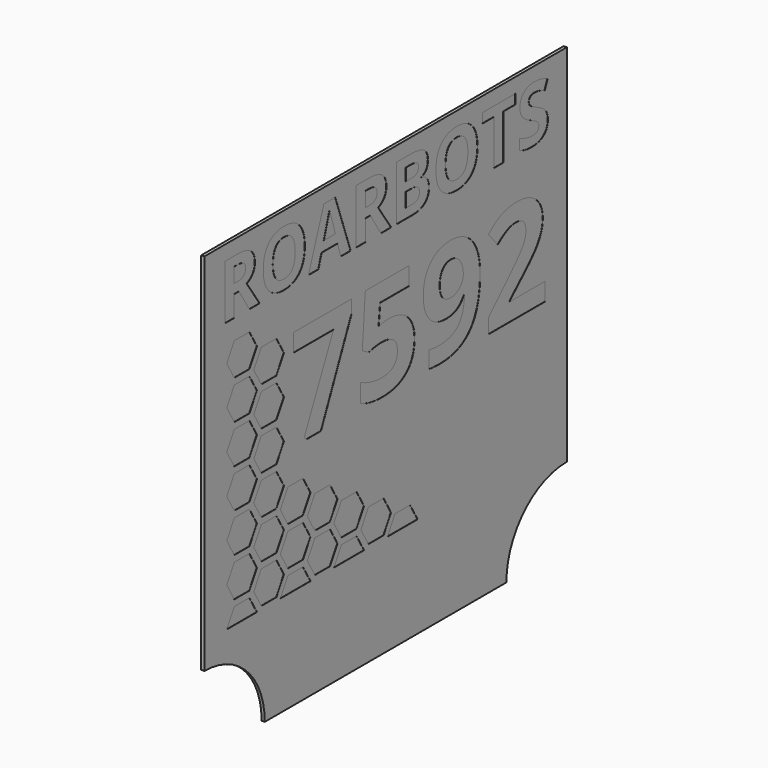
from build123d import *

# Parameters (mm, degrees)
F1_DEPTH     = 3.175
F2_TEXT_SIZE = 77.282099
F3_DEPTH     = 0.254


# Not quite as in the source:
# - Text() gives the source's letters only with a copy of the font that has no kerning and outlines rounded to 1/6400 em; it was checked with that copy


with BuildPart() as f1:
    # F0 (on Right) → F1 (new body)
    with BuildSketch(Plane.YZ):
        with BuildLine():
            ThreePointArc((-228.6, -146.05), (-174.718463, -168.368463), (-152.4, -222.25))
            Line((-152.4, -222.25), (152.4, -222.25))
            ThreePointArc((152.4, -222.25), (174.718463, -168.368463), (228.6, -146.05))
            Line((228.6, -146.05), (228.6, 222.25))
            Line((228.6, 222.25), (-228.6, 222.25))
            Line((-228.6, 222.25), (-228.6, -146.05))
        make_face()
    extrude(amount=F1_DEPTH)

    # F2 (on face) → F3 (cut)
    with BuildSketch(Plane.YZ.offset(3.175)):
        Polygon((-190.800815, -104.152216), (-200.325815, -120.65), (-181.275815, -120.65), (-166.988315, -112.401108), (-171.750815, -104.152216), align=None)
        Polygon((-166.988315, -112.401108), (-181.275815, -120.65), (-162.225815, -120.65), align=None)
        Polygon((-166.251553, -100.977216), (-161.489053, -109.226108), (-156.726553, -117.475), (-137.676553, -117.475), (-128.151553, -100.977216), (-137.676553, -84.479432), (-156.726553, -84.479432), align=None)
        Polygon((-123.236815, -104.152216), (-132.761815, -120.65), (-94.661815, -120.65), (-104.186815, -104.152216), align=None)
        Polygon((-89.162553, -117.475), (-70.112553, -117.475), (-60.587553, -100.977216), (-70.112553, -84.479432), (-89.162553, -84.479432), (-98.687553, -100.977216), align=None)
        Polygon((-55.672815, -104.152216), (-65.197815, -120.65), (-27.097815, -120.65), (-36.622815, -104.152216), align=None)
        Polygon((-21.598553, -117.475), (-2.548553, -117.475), (6.976447, -100.977216), (-2.548553, -84.479432), (-21.598553, -84.479432), (-31.123553, -100.977216), align=None)
        Polygon((2.366185, -120.65), (40.466185, -120.65), (30.941185, -104.152216), (11.891185, -104.152216), align=None)
        Polygon((-65.197815, -81.28), (-55.672815, -97.777784), (-36.622815, -97.777784), (-27.097815, -81.28), (-36.622815, -64.782216), (-55.672815, -64.782216), align=None)
        Polygon((-98.687553, -61.607216), (-89.162553, -78.105), (-70.112553, -78.105), (-60.587553, -61.607216), (-70.112553, -45.109432), (-89.162553, -45.109432), align=None)
        Polygon((-123.236815, -25.412216), (-132.761815, -41.91), (-123.236815, -58.407784), (-104.186815, -58.407784), (-94.661815, -41.91), (-104.186815, -25.412216), align=None)
        Polygon((-156.726553, -38.735), (-137.676553, -38.735), (-128.151553, -22.237216), (-137.676553, -5.739432), (-156.726553, -5.739432), (-166.251553, -22.237216), align=None)
        Polygon((-156.726553, 0.635), (-137.676553, 0.635), (-128.151553, 17.132784), (-137.676553, 33.630568), (-156.726553, 33.630568), (-166.251553, 17.132784), align=None)
        Polygon((-156.726553, 40.005), (-137.676553, 40.005), (-128.151553, 56.502784), (-137.676553, 73.000568), (-156.726553, 73.000568), (-166.251553, 56.502784), align=None)
        Polygon((-156.726553, 79.375), (-137.676553, 79.375), (-128.151553, 95.872784), (-137.676553, 112.370568), (-156.726553, 112.370568), (-166.251553, 95.872784), align=None)
        Polygon((-171.750815, 99.072216), (-162.225815, 115.57), (-171.750815, 132.067784), (-190.800815, 132.067784), (-200.325815, 115.57), (-190.800815, 99.072216), align=None)
        Polygon((-171.750815, 59.702216), (-162.225815, 76.2), (-171.750815, 92.697784), (-190.800815, 92.697784), (-200.325815, 76.2), (-190.800815, 59.702216), align=None)
        Polygon((-171.750815, 20.332216), (-162.225815, 36.83), (-171.750815, 53.327784), (-190.800815, 53.327784), (-200.325815, 36.83), (-190.800815, 20.332216), align=None)
        Polygon((-171.750815, -19.037784), (-162.225815, -2.54), (-171.750815, 13.957784), (-190.800815, 13.957784), (-200.325815, -2.54), (-190.800815, -19.037784), align=None)
        Polygon((-171.750815, -58.407784), (-162.225815, -41.91), (-171.750815, -25.412216), (-190.800815, -25.412216), (-200.325815, -41.91), (-190.800815, -58.407784), align=None)
        Polygon((-171.750815, -97.777784), (-162.225815, -81.28), (-171.750815, -64.782216), (-190.800815, -64.782216), (-200.325815, -81.28), (-190.800815, -97.777784), align=None)
        Polygon((-156.726553, -78.105), (-137.676553, -78.105), (-128.151553, -61.607216), (-137.676553, -45.109432), (-156.726553, -45.109432), (-166.251553, -61.607216), align=None)
        Polygon((-123.236815, -64.782216), (-132.761815, -81.28), (-123.236815, -97.777784), (-104.186815, -97.777784), (-94.661815, -81.28), (-104.186815, -64.782216), align=None)
        Polygon((-89.007763, 40.005), (-102.3683, 10.808023), (-100.384996, 7.37284), (-93.052647, 7.37284), (-98.687553, 17.132784), (-89.162553, 33.630568), (-70.112553, 33.630568), (-69.995235, 33.427367), (-42.885315, 95.491512), (-42.885315, 109.012249), (-68.173627, 109.012249), (-60.587553, 95.872784), (-70.112553, 79.375), (-70.992051, 79.375), (-73.908991, 73.000568), (-70.112553, 73.000568), (-60.587553, 56.502784), (-70.112553, 40.005), align=None)
        Polygon((-98.687553, 17.132784), (-93.052647, 7.37284), (-81.375979, 7.37284), (-69.995235, 33.427367), (-70.112553, 33.630568), (-89.162553, 33.630568), align=None)
        Polygon((-73.908991, 73.000568), (-89.007763, 40.005), (-70.112553, 40.005), (-60.587553, 56.502784), (-70.112553, 73.000568), align=None)
        Polygon((-65.716872, 90.902926), (-70.992051, 79.375), (-70.112553, 79.375), (-60.587553, 95.872784), (-68.173627, 109.012249), (-91.10148, 109.012249), (-98.687553, 95.872784), (-95.818205, 90.902926), align=None)
        Polygon((-103.150553, 90.902926), (-95.818205, 90.902926), (-98.687553, 95.872784), (-91.10148, 109.012249), (-98.447934, 109.012249), (-104.186815, 99.072216), (-115.901748, 99.072216), (-115.901748, 92.697784), (-104.186815, 92.697784), align=None)
        Polygon((-104.186815, 99.072216), (-98.447934, 109.012249), (-115.901748, 109.012249), (-115.901748, 99.072216), align=None)
        Polygon((-115.901748, 90.902926), (-103.150553, 90.902926), (-104.186815, 92.697784), (-115.901748, 92.697784), align=None)
        with BuildLine():
            add(Edge.make_bspline(
                [(4.381576, 72.392659), (19.127421, 72.392659), (27.870237, 64.106475)],
                knots=[0, 0, 0, 1, 1, 1], degree=2))
            add(Edge.make_bspline(
                [(-6.132077, 71.412573), (-1.877611, 72.392659), (4.381576, 72.392659)],
                knots=[0, 0, 0, 1, 1, 1], degree=2))
            Line((-6.132077, 71.412573), (-8.560018, 70.92253))
            Line((-8.560018, 70.92253), (-6.688944, 90.902926))
            Line((-6.688944, 90.902926), (29.641074, 90.902926))
            Line((29.641074, 90.902926), (29.641074, 109.145897))
            Line((29.641074, 109.145897), (-25.555607, 109.145897))
            Line((-25.555607, 109.145897), (-29.386853, 57.290419))
            Line((-29.386853, 57.290419), (-20.811098, 52.679559))
            add(Edge.make_bspline(
                [(-13.571824, 54.261062), (-18.026761, 53.525997), (-20.811098, 52.679559)],
                knots=[0, 0, 0, 1, 1, 1], degree=2))
            add(Edge.make_bspline(
                [(-5.441562, 54.996126), (-9.116886, 54.996126), (-13.571824, 54.261062)],
                knots=[0, 0, 0, 1, 1, 1], degree=2))
            add(Edge.make_bspline(
                [(14.962054, 39.604316), (14.962054, 54.996126), (-5.441562, 54.996126)],
                knots=[0, 0, 0, 1, 1, 1], degree=2))
            add(Edge.make_bspline(
                [(-4.751046, 23.455166), (14.962054, 23.455166), (14.962054, 39.604316)],
                knots=[0, 0, 0, 1, 1, 1], degree=2))
            add(Edge.make_bspline(
                [(-18.594766, 25.303965), (-11.27753, 23.455166), (-4.751046, 23.455166)],
                knots=[0, 0, 0, 1, 1, 1], degree=2))
            add(Edge.make_bspline(
                [(-31.391575, 30.070749), (-25.912002, 27.152764), (-18.594766, 25.303965)],
                knots=[0, 0, 0, 1, 1, 1], degree=2))
            Line((-31.391575, 30.070749), (-31.391575, 11.471383))
            add(Edge.make_bspline(
                [(-3.971432, 5.969534), (-20.96702, 5.969534), (-31.391575, 11.471383)],
                knots=[0, 0, 0, 1, 1, 1], degree=2))
            add(Edge.make_bspline(
                [(26.099399, 15.168981), (15.585745, 5.969534), (-3.971432, 5.969534)],
                knots=[0, 0, 0, 1, 1, 1], degree=2))
            add(Edge.make_bspline(
                [(36.613052, 41.408566), (36.613052, 24.368428), (26.099399, 15.168981)],
                knots=[0, 0, 0, 1, 1, 1], degree=2))
            add(Edge.make_bspline(
                [(27.870237, 64.106475), (36.613052, 55.82029), (36.613052, 41.408566)],
                knots=[0, 0, 0, 1, 1, 1], degree=2))
        make_face()
        with BuildLine():
            add(Edge.make_bspline(
                [(119.430349, 65.710252), (119.430349, 35.639421), (106.767188, 20.804478)],
                knots=[0, 0, 0, 1, 1, 1], degree=2))
            add(Edge.make_bspline(
                [(114.908587, 89.688956), (119.430349, 79.631933), (119.430349, 65.710252)],
                knots=[0, 0, 0, 1, 1, 1], degree=2))
            add(Edge.make_bspline(
                [(101.93358, 105.036217), (110.386825, 99.745978), (114.908587, 89.688956)],
                knots=[0, 0, 0, 1, 1, 1], degree=2))
            add(Edge.make_bspline(
                [(82.187067, 110.326456), (93.480335, 110.326456), (101.93358, 105.036217)],
                knots=[0, 0, 0, 1, 1, 1], degree=2))
            add(Edge.make_bspline(
                [(56.894157, 100.8263), (66.19384, 110.326456), (82.187067, 110.326456)],
                knots=[0, 0, 0, 1, 1, 1], degree=2))
            add(Edge.make_bspline(
                [(47.594474, 74.954248), (47.594474, 91.326145), (56.894157, 100.8263)],
                knots=[0, 0, 0, 1, 1, 1], degree=2))
            add(Edge.make_bspline(
                [(55.256968, 51.265116), (47.594474, 59.785185), (47.594474, 74.954248)],
                knots=[0, 0, 0, 1, 1, 1], degree=2))
            add(Edge.make_bspline(
                [(76.217451, 42.745047), (62.919461, 42.745047), (55.256968, 51.265116)],
                knots=[0, 0, 0, 1, 1, 1], degree=2))
            add(Edge.make_bspline(
                [(89.437479, 45.384598), (84.14724, 42.745047), (76.217451, 42.745047)],
                knots=[0, 0, 0, 1, 1, 1], degree=2))
            add(Edge.make_bspline(
                [(98.759437, 54.572907), (94.727718, 48.024149), (89.437479, 45.384598)],
                knots=[0, 0, 0, 1, 1, 1], degree=2))
            Line((98.759437, 54.572907), (99.605875, 54.572907))
            add(Edge.make_bspline(
                [(95.351409, 35.873305), (99.049008, 42.655948), (99.605875, 54.572907)],
                knots=[0, 0, 0, 1, 1, 1], degree=2))
            add(Edge.make_bspline(
                [(84.69297, 25.927656), (91.653811, 29.090662), (95.351409, 35.873305)],
                knots=[0, 0, 0, 1, 1, 1], degree=2))
            add(Edge.make_bspline(
                [(66.95118, 22.76465), (77.73213, 22.76465), (84.69297, 25.927656)],
                knots=[0, 0, 0, 1, 1, 1], degree=2))
            add(Edge.make_bspline(
                [(54.7001, 24.212505), (60.558344, 22.76465), (66.95118, 22.76465)],
                knots=[0, 0, 0, 1, 1, 1], degree=2))
            Line((54.7001, 24.212505), (54.7001, 6.949621))
            add(Edge.make_bspline(
                [(68.421309, 5.969534), (59.355511, 5.969534), (54.7001, 6.949621)],
                knots=[0, 0, 0, 1, 1, 1], degree=2))
            add(Edge.make_bspline(
                [(106.767188, 20.804478), (94.104026, 5.969534), (68.421309, 5.969534)],
                knots=[0, 0, 0, 1, 1, 1], degree=2))
        make_face()
        with BuildLine():
            add(Edge.make_bspline(
                [(82.610287, 93.063571), (75.92788, 93.063571), (72.174594, 88.463848)],
                knots=[0, 0, 0, 1, 1, 1], degree=2))
            add(Edge.make_bspline(
                [(93.714219, 87.350113), (89.359518, 93.063571), (82.610287, 93.063571)],
                knots=[0, 0, 0, 1, 1, 1], degree=2))
            add(Edge.make_bspline(
                [(98.068921, 73.372745), (98.068921, 81.636655), (93.714219, 87.350113)],
                knots=[0, 0, 0, 1, 1, 1], degree=2))
            add(Edge.make_bspline(
                [(93.402374, 63.516195), (98.068921, 67.804073), (98.068921, 73.372745)],
                knots=[0, 0, 0, 1, 1, 1], degree=2))
            add(Edge.make_bspline(
                [(82.187067, 59.228317), (88.735826, 59.228317), (93.402374, 63.516195)],
                knots=[0, 0, 0, 1, 1, 1], degree=2))
            add(Edge.make_bspline(
                [(71.829337, 63.549607), (75.237364, 59.228317), (82.187067, 59.228317)],
                knots=[0, 0, 0, 1, 1, 1], degree=2))
            add(Edge.make_bspline(
                [(68.421309, 75.243819), (68.421309, 67.870897), (71.829337, 63.549607)],
                knots=[0, 0, 0, 1, 1, 1], degree=2))
            add(Edge.make_bspline(
                [(72.174594, 88.463848), (68.421309, 83.864124), (68.421309, 75.243819)],
                knots=[0, 0, 0, 1, 1, 1], degree=2))
        make_face(mode=Mode.SUBTRACT)
        with BuildLine():
            Line((130.07765, 7.37284), (201.223009, 7.37284))
            Line((201.223009, 7.37284), (201.223009, 25.482163))
            Line((201.223009, 25.482163), (156.874102, 25.482163))
            Line((156.874102, 25.482163), (156.874102, 26.439974))
            Line((156.874102, 26.439974), (169.97162, 38.757878))
            add(Edge.make_bspline(
                [(188.236865, 57.212458), (183.046862, 50.741661), (169.97162, 38.757878)],
                knots=[0, 0, 0, 1, 1, 1], degree=2))
            add(Edge.make_bspline(
                [(195.899358, 69.842207), (193.426868, 63.683255), (188.236865, 57.212458)],
                knots=[0, 0, 0, 1, 1, 1], degree=2))
            add(Edge.make_bspline(
                [(198.371849, 83.039961), (198.371849, 76.001159), (195.899358, 69.842207)],
                knots=[0, 0, 0, 1, 1, 1], degree=2))
            add(Edge.make_bspline(
                [(194.328993, 97.373724), (198.371849, 91.103398), (198.371849, 83.039961)],
                knots=[0, 0, 0, 1, 1, 1], degree=2))
            add(Edge.make_bspline(
                [(182.980038, 107.1189), (190.286137, 103.644049), (194.328993, 97.373724)],
                knots=[0, 0, 0, 1, 1, 1], degree=2))
            add(Edge.make_bspline(
                [(166.140373, 110.593752), (175.67394, 110.593752), (182.980038, 107.1189)],
                knots=[0, 0, 0, 1, 1, 1], degree=2))
            add(Edge.make_bspline(
                [(153.053993, 109.168172), (158.901099, 110.593752), (166.140373, 110.593752)],
                knots=[0, 0, 0, 1, 1, 1], degree=2))
            add(Edge.make_bspline(
                [(142.261906, 105.103041), (147.206887, 107.742592), (153.053993, 109.168172)],
                knots=[0, 0, 0, 1, 1, 1], degree=2))
            add(Edge.make_bspline(
                [(129.810354, 96.04838), (137.316924, 102.46349), (142.261906, 105.103041)],
                knots=[0, 0, 0, 1, 1, 1], degree=2))
            Line((129.810354, 96.04838), (141.504566, 82.193523))
            add(Edge.make_bspline(
                [(153.131954, 89.92284), (147.563282, 87.205328), (141.504566, 82.193523)],
                knots=[0, 0, 0, 1, 1, 1], degree=2))
            add(Edge.make_bspline(
                [(164.603419, 92.640352), (158.700627, 92.640352), (153.131954, 89.92284)],
                knots=[0, 0, 0, 1, 1, 1], degree=2))
            add(Edge.make_bspline(
                [(173.624669, 89.644406), (170.238916, 92.640352), (164.603419, 92.640352)],
                knots=[0, 0, 0, 1, 1, 1], degree=2))
            add(Edge.make_bspline(
                [(177.010421, 80.522921), (177.010421, 86.648461), (173.624669, 89.644406)],
                knots=[0, 0, 0, 1, 1, 1], degree=2))
            add(Edge.make_bspline(
                [(175.473468, 72.593131), (177.010421, 76.424378), (177.010421, 80.522921)],
                knots=[0, 0, 0, 1, 1, 1], degree=2))
            add(Edge.make_bspline(
                [(170.461663, 64.273535), (173.936514, 68.761885), (175.473468, 72.593131)],
                knots=[0, 0, 0, 1, 1, 1], degree=2))
            add(Edge.make_bspline(
                [(155.626719, 48.157797), (166.986811, 59.785185), (170.461663, 64.273535)],
                knots=[0, 0, 0, 1, 1, 1], degree=2))
            Line((155.626719, 48.157797), (130.07765, 22.341431))
            Line((130.07765, 22.341431), (130.07765, 7.37284))
        make_face()
        with Locations((-209.790711, 152.24044)):
            Text('ROARBOTS', F2_TEXT_SIZE, font='Open Sans', font_style=FontStyle.BOLD, text_align=(TextAlign.LEFT, TextAlign.BOTTOM))
    extrude(amount=-F3_DEPTH, mode=Mode.SUBTRACT)


solid = f1.part
